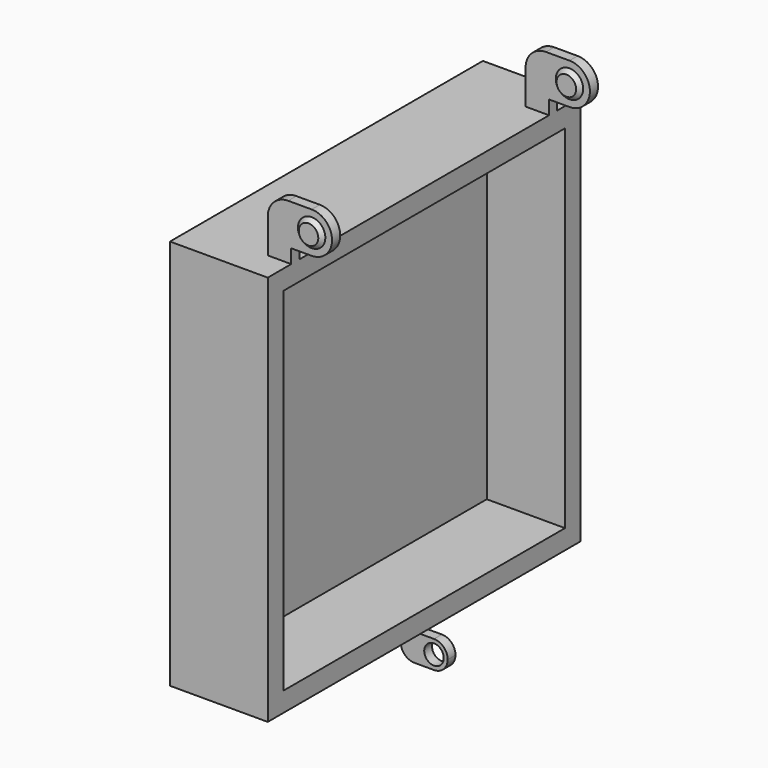
from build123d import *

# Parameters (mm, degrees)
F0_W      = 127
F0_H      = 127
F0_W_2    = 114.3
F0_H_2    = 114.3
F1_DEPTH  = 25.4
F2_W      = 127
F2_H      = 127
F3_DEPTH  = 6.35
F4_W      = 20.8788
F4_H      = 3.302
F5_DEPTH  = 17.78
F6_R      = 6.6294
F8_DEPTH  = 6.35
F9_R      = 6.6294
F10_R     = 4.445
F11_DEPTH = 1.27
F12_R     = 4.445
F13_DEPTH = 1.27
F14_SIZE  = 1.26999
F15_W     = 15.24
F15_H     = 8.89
F16_DEPTH = 1.5875
F17_R     = 4.44499
F18_R     = 3.175
F19_DEPTH = 25.4


# Not quite as in the source:
# - a fillet or chamfer is up to 0.001 mm smaller than in the source, because OpenCascade refuses the exact size
# - a pattern or mirror of a feature is missing from the dataset's text; its kind, count and spacing are read off the source's solid


with BuildPart() as f1:
    # F0 (on Right) → F1 (new body)
    with BuildSketch(Plane.YZ):
        Rectangle(F0_W, F0_H)
        Rectangle(F0_W_2, F0_H_2, mode=Mode.SUBTRACT)
    extrude(amount=F1_DEPTH)

    # F2 (on Right) → F3 (join)
    with BuildSketch(Plane.YZ):
        Rectangle(F2_W, F2_H)
    extrude(amount=-F3_DEPTH)

    # F4 (on face) → F5 (join)
    with BuildSketch(Plane.XY.offset(63.5)):
        with Locations((28.2194, -52.324)):
            Rectangle(F4_W, F4_H)
    f5 = extrude(amount=F5_DEPTH)

    # F5_copies: F5 across plane
    add(f5.mirror(Plane.ZX))

    # F6
    f6_edges = [f1.edges().sort_by_distance(p)[0] for p in [
        (38.6588, -52.324, 81.28),
    ]]
    fillet(f6_edges, radius=F6_R)

    # F7 (on face) → F8 (cut)
    with BuildSketch(Plane.XZ.offset(53.975)):
        with BuildLine():
            ThreePointArc((32.0294, 81.28), (38.6588, 74.6506), (32.0294, 68.0212))
            Line((32.0294, 68.0212), (25.4, 68.0212))
            Line((25.4, 68.0212), (25.4, 63.5))
            Line((25.4, 63.5), (41.4029210806, 57.3826394975))
            Line((41.4029210806, 57.3826394975), (43.7219925225, 87.7940133214))
            Line((43.7219925225, 87.7940133214), (32.0294, 81.28))
        make_face()
    f8 = extrude(amount=-F8_DEPTH, mode=Mode.SUBTRACT)

    # F8_copies: F8 across plane
    add(f8.mirror(Plane.ZX), mode=Mode.SUBTRACT)

    # F9
    f9_edges = [f1.edges().sort_by_distance(p)[0] for p in [
        (17.78, -52.324, 81.28),
        (17.78, 52.324, 81.28),
    ]]
    fillet(f9_edges, radius=F9_R)

    # F10 (on face) → F11 (join)
    with BuildSketch(Plane.XZ.offset(53.975)):
        with Locations((32.0294, 74.6506)):
            Circle(F10_R)
    f11 = extrude(amount=F11_DEPTH)

    # F11_copies: F11 across plane
    add(f11.mirror(Plane.ZX))

    # F12 (on face) → F13 (join)
    with BuildSketch(Plane(origin=(0, -50.673, 0), x_dir=(-1, 0, 0), z_dir=(0, 1, 0))):
        with Locations((-32.0294, 74.6506)):
            Circle(F12_R)
    f13 = extrude(amount=F13_DEPTH)

    # F13_copies: F13 across plane
    add(f13.mirror(Plane.ZX))

    # F14 (size 1.27 in the source; OpenCascade refuses exactly that, so slightly less here)
    f14_edges = [f1.edges().sort_by_distance(p)[0] for p in [
        (27.5844, -55.245, 74.6506),
        (36.4744, -49.403, 74.6506),
        (27.5844, 55.245, 74.6506),
        (36.4744, 49.403, 74.6506),
    ]]
    chamfer(f14_edges, length=F14_SIZE)

    # F15 (on Front) → F16 (join, symmetric)
    with BuildSketch(Plane.XZ):
        with Locations((26.67, -67.945)):
            Rectangle(F15_W, F15_H)
    extrude(amount=F16_DEPTH, both=True)

    # F17 (radius 4.445 in the source; OpenCascade refuses exactly that, so slightly less here)
    f17_edges = [f1.edges().sort_by_distance(p)[0] for p in [
        (34.29, 0, -63.5),
        (34.29, 0, -72.39),
        (19.05, 0, -72.39),
    ]]
    fillet(f17_edges, radius=F17_R)

    # F18 (on face) → F19 (cut)
    with BuildSketch(Plane(origin=(0, 1.5875, 0), x_dir=(-1, 0, 0), z_dir=(0, 1, 0))):
        with Locations((-29.845, -67.945)):
            Circle(F18_R)
    extrude(amount=-F19_DEPTH, mode=Mode.SUBTRACT)


solid = f1.part
